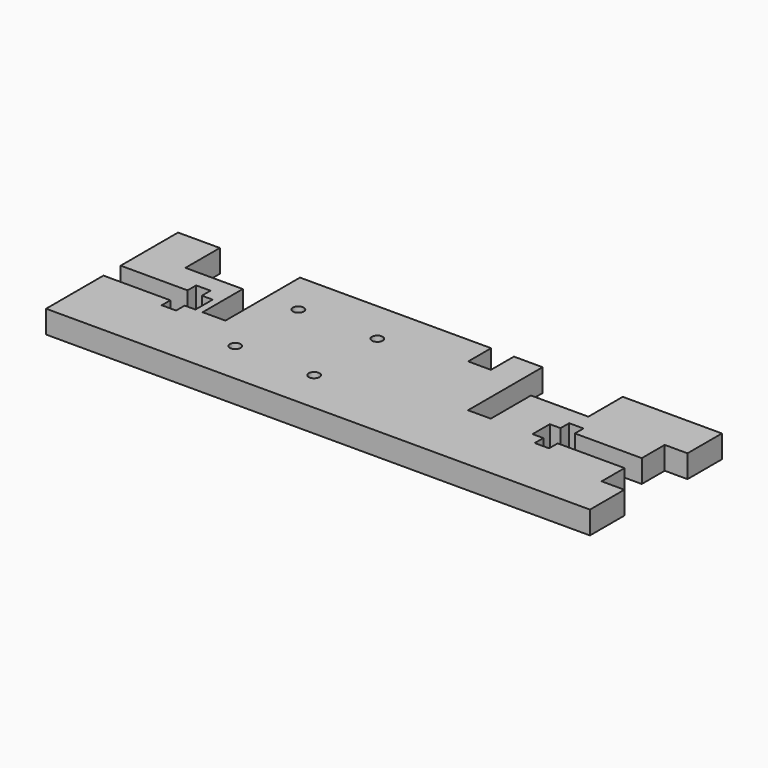
from build123d import *

# Parameters (mm, degrees)
F0_R     = 0.75
F0_W     = 3.175
F0_H     = 6
F1_DEPTH = 3.175


# Not quite as in the source:
# - a length typed as a fraction of an inch, garbled in the dataset ("3 / 203.2 mm" for 3/8 in), is restored


with BuildPart() as f1:
    # F0 (on Top) → F1 (new body)
    with BuildSketch(Plane.XY):
        Polygon((21.0674113333, 24.2020648569), (21.0674113333, 27.2020648569), (22.5674113333, 27.2020648569), (22.5674113333, 28.7020648569), (24.5674113333, 28.7020648569), (24.5674113333, 27.2020648569), (33.8924113333, 27.2020648569), (33.8924113333, 31.2020648569), (33.8924113333, 37.2020648569), (23.2424113333, 37.2020648569), (23.2424113333, 31.2020648569), (15.2424113333, 31.2020648569), (15.2424113333, 24.2020648569), (12.0674113333, 24.2020648569), (12.0674113333, 37.2020648569), (8.0674113333, 37.2020648569), (8.0674113333, 33.2020648569), (4.8924113333, 33.2020648569), (4.8924113333, 37.2020648569), (-21.7575886667, 37.2020648569), (-21.7575886667, 24.2020648569), (-24.9325886667, 24.2020648569), (-24.9325886667, 31.2020648569), (-32.9325886667, 31.2020648569), (-32.9325886667, 37.2020648569), (-38.7575886667, 37.2020648569), (-38.7575886667, 31.2020648569), (-38.7575886667, 27.2020648569), (-29.4325886667, 27.2020648569), (-29.4325886667, 28.7020648569), (-27.4325886667, 28.7020648569), (-27.4325886667, 27.2020648569), (-25.9325886667, 27.2020648569), (-25.9325886667, 24.2020648569), (-27.4325886667, 24.2020648569), (-27.4325886667, 22.7020648569), (-29.4325886667, 22.7020648569), (-29.4325886667, 24.2020648569), (-38.7575886667, 24.2020648569), (-38.7575886667, 20.2020648569), (-38.7575886667, 14.2020648569), (33.8924113333, 14.2020648569), (33.8924113333, 20.2020648569), (33.8924113333, 24.2020648569), (24.5674113333, 24.2020648569), (24.5674113333, 22.7020648569), (22.5674113333, 22.7020648569), (22.5674113333, 24.2020648569), align=None)
        with Locations((-17.1825886667, 20.2020648569)):
            Circle(F0_R, mode=Mode.SUBTRACT)
        with Locations((-6.1825886667, 20.2020648569)):
            Circle(F0_R, mode=Mode.SUBTRACT)
        with Locations((-17.1825886667, 31.2020648569)):
            Circle(F0_R, mode=Mode.SUBTRACT)
        with Locations((-6.1825886667, 31.2020648569)):
            Circle(F0_R, mode=Mode.SUBTRACT)
        with Locations((35.4799113333, 34.2020648569)):
            Rectangle(F0_W, F0_H)
        with Locations((35.4799113333, 17.2020648569)):
            Rectangle(F0_W, F0_H)
    extrude(amount=F1_DEPTH)


solid = f1.part
